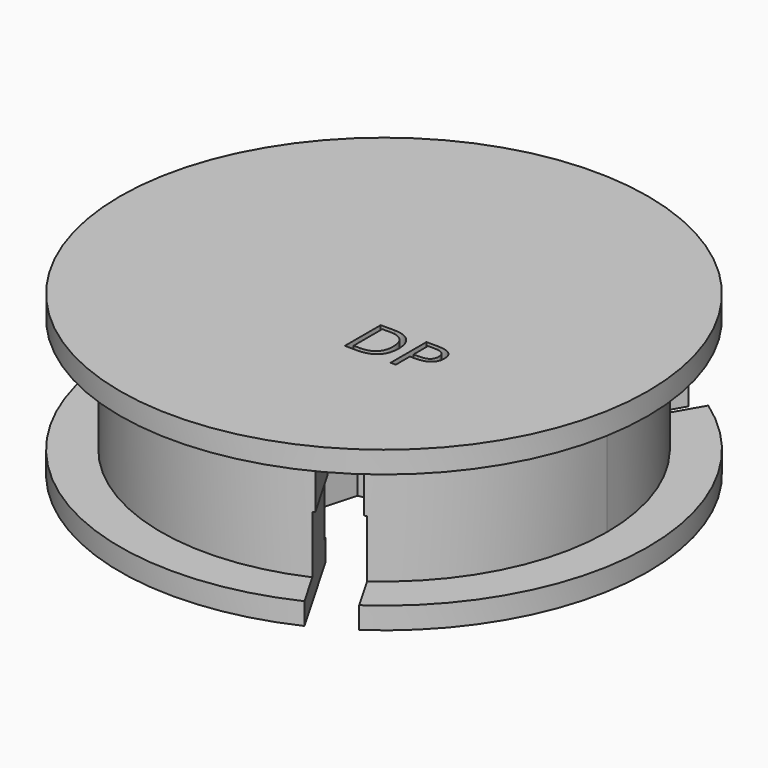
from build123d import *

# Parameters (mm, degrees)
F1_DEPTH     = 25.4
F2_W         = 17.2924827784
F2_H         = 3.4843063913
F5_DEPTH     = 5.08
F7_TEXT_SIZE = 10.0370975108
F8_DEPTH     = 25.4
F10_DEPTH    = 12.7


# Not quite as in the source:
# - Text() gives the source's letters only with a copy of the font that has no kerning and outlines rounded to 1/6400 em; it was checked with that copy


with BuildPart() as f1:
    # F0 (on Top) → F1 (new body)
    with BuildSketch(Plane.XY):
        with BuildLine():
            ThreePointArc((-35.5599578277, -2.9174165863), (-17.9904863515, -30.8117562155), (14.9374873191, -32.402058466))
            Line((14.9374873191, -32.402058466), (9.9298087673, -23.7285047862))
            ThreePointArc((9.9298087673, -23.7285047862), (2.9868714083, -25.5484175779), (-4.1886279773, -25.3790944916))
            ThreePointArc((-4.1886279773, -25.3790944916), (-6.9308146444, -24.7710889932), (-9.5903600923, -23.867719515))
            ThreePointArc((-9.5903600923, -23.867719515), (-20.458573278, -15.591338011), (-25.5564418886, -2.9174165863))
            Line((-25.5564418886, -2.9174165863), (-35.5599578277, -2.9174165863))
        make_face()
        with BuildLine():
            Line((10.2516640672, 23.591236199), (15.2534220367, 32.2545351294))
            ThreePointArc((15.2534220367, 32.2545351294), (-17.6885204421, 30.9860963145), (-35.529749426, 3.2647857459))
            Line((-35.529749426, 3.2647857459), (-25.5143923223, 3.2647857459))
            ThreePointArc((-25.5143923223, 3.2647857459), (-23.6190143531, 10.1875022715), (-19.8846265661, 16.3170054811))
            ThreePointArc((-19.8846265661, 16.3170054811), (-17.9869850253, 18.3878060476), (-15.8748713842, 20.2393552289))
            ThreePointArc((-15.8748713842, 20.2393552289), (-3.2732081575, 25.5133131894), (10.2516640672, 23.591236199))
        make_face()
        with BuildLine():
            ThreePointArc((20.306535791, -29.3371185431), (31.603382715, -16.5604384366), (35.6794327343, 0))
            ThreePointArc((35.6794327343, 0), (31.6839245591, 16.4058174065), (20.5922621069, 29.1372727201))
            Line((20.5922621069, 29.1372727201), (15.584583555, 20.4637190403))
            ThreePointArc((15.584583555, 20.4637190403), (20.6321429448, 15.3609153064), (24.0732545434, 9.0620890104))
            ThreePointArc((24.0732545434, 9.0620890104), (24.9177996697, 6.3832829456), (25.4652314765, 3.6283642861))
            ThreePointArc((25.4652314765, 3.6283642861), (25.6580445053, 1.8187340953), (25.722422933, 0))
            ThreePointArc((25.722422933, 0), (22.9708403151, -11.5751257774), (15.3047778215, -20.6738196128))
            Line((15.3047778215, -20.6738196128), (20.306535791, -29.3371185431))
        make_face()
        with BuildLine():
            Line((-2.3523073549, 6.2661422281), (-15.8748713842, 20.2393552289))
            ThreePointArc((-15.8748713842, 20.2393552289), (-17.9869850253, 18.3878060476), (-19.8846265661, 16.3170054811))
            Line((-19.8846265661, 16.3170054811), (-6.2411793261, 2.4177611409))
            ThreePointArc((-6.2411793261, 2.4177611409), (-4.7079201971, 4.7574547536), (-2.3523073549, 6.2661422281))
        make_face()
        with BuildLine():
            ThreePointArc((25.4652314765, 3.6283642861), (24.9177996697, 6.3832829456), (24.0732545434, 9.0620890104))
            Line((24.0732545434, 9.0620890104), (5.2144322314, 4.1961392755))
            ThreePointArc((5.2144322314, 4.1961392755), (6.3126350211, 2.2245285806), (6.6931224638, 0))
            ThreePointArc((6.6931224638, 0), (6.6705016295, -0.54981481), (6.6027920307, -1.0959131872))
            Line((6.6027920307, -1.0959131872), (25.4652314765, 3.6283642861))
        make_face()
        with BuildLine():
            ThreePointArc((-9.5903600923, -23.867719515), (-6.9308146444, -24.7710889932), (-4.1886279773, -25.3790944916))
            Line((-4.1886279773, -25.3790944916), (1.0267470947, -6.6139004164))
            ThreePointArc((1.0267470947, -6.6139004164), (-1.7661165754, -6.4559058665), (-4.2504846758, -5.1702290409))
            Line((-4.2504846758, -5.1702290409), (-9.5903600923, -23.867719515))
        make_face()
        with BuildLine():
            ThreePointArc((6.6931224638, 0), (6.3126350211, 2.2245285806), (5.2144322314, 4.1961392755))
            ThreePointArc((5.2144322314, 4.1961392755), (1.7661165754, 6.4559058665), (-2.3523073549, 6.2661422281))
            ThreePointArc((-2.3523073549, 6.2661422281), (-4.7079201971, 4.7574547536), (-6.2411793261, 2.4177611409))
            ThreePointArc((-6.2411793261, 2.4177611409), (-6.4740367725, -1.6984511129), (-4.2504846758, -5.1702290409))
            ThreePointArc((-4.2504846758, -5.1702290409), (-1.7661165754, -6.4559058665), (1.0267470947, -6.6139004164))
            ThreePointArc((1.0267470947, -6.6139004164), (4.7079201971, -4.7574547536), (6.6027920307, -1.0959131872))
            ThreePointArc((6.6027920307, -1.0959131872), (6.6705016295, -0.54981481), (6.6931224638, 0))
        make_face()
    extrude(amount=F1_DEPTH)

    # F2 (on Front) → F3 (revolve)
    with BuildSketch(Plane.XZ):
        Polygon((-24.9063391238, 21.9382257201), (0, 21.9382257201), (0, 25.4225321114), (-42.1988219023, 25.4225321114), (-42.1988219023, 21.9382257201), align=None)
        with Locations((-33.5525805131, 1.7421531957)):
            Rectangle(F2_W, F2_H)
    revolve(axis=Axis((0, 0, 18.905589357), (0, 0, 1)))

    # F4 (on Top) → F5 (cut)
    with BuildSketch(Plane.XY):
        Polygon((-46.8445643783, -3.2262096647), (-23.0996608734, -3.2262096647), (-22.841565311, 3.2262096647), (-47.6188547909, 3.2262096647), align=None)
        Polygon((26.2162617167, -38.9554779484), (14.3438099643, -18.3917883028), (8.6268031279, -21.3944806538), (21.0154478679, -42.8522427804), align=None)
        Polygon((20.6283026616, 42.1816876131), (8.7558509091, 21.6179979675), (14.2147621831, 18.1682709891), (26.603406923, 39.6260331157), align=None)
    extrude(amount=-F5_DEPTH, mode=Mode.SUBTRACT)

    # F7 (on offset) → F8 (cut)
    with BuildSketch(Plane.XY.offset(21.844)):
        with Locations((4.0004982147, -14.0662742779)):
            Text('DP', F7_TEXT_SIZE, font='Open Sans', text_align=(TextAlign.LEFT, TextAlign.BOTTOM))
    extrude(amount=F8_DEPTH, mode=Mode.SUBTRACT)

    # F9 (on Top) → F10 (cut)
    with BuildSketch(Plane.XY):
        Polygon((14.5824700594, -18.7120158225), (8.3881476894, -21.8091774732), (23.8739531487, -48.6512444913), (31.8749509752, -48.6512444913), align=None)
        Polygon((8.9138460286, 21.9847974326), (14.6932278827, 18.1689377263), (30.1962370809, 45.0010721612), (26.1957381676, 51.9301395346), align=None)
        Polygon((-23.496316088, -3.2727816101), (-23.0813755721, 3.6402397469), (-54.0701902296, 3.6501723301), (-58.0706891428, -3.2788950432), align=None)
    extrude(amount=F10_DEPTH, mode=Mode.SUBTRACT)


solid = f1.part
